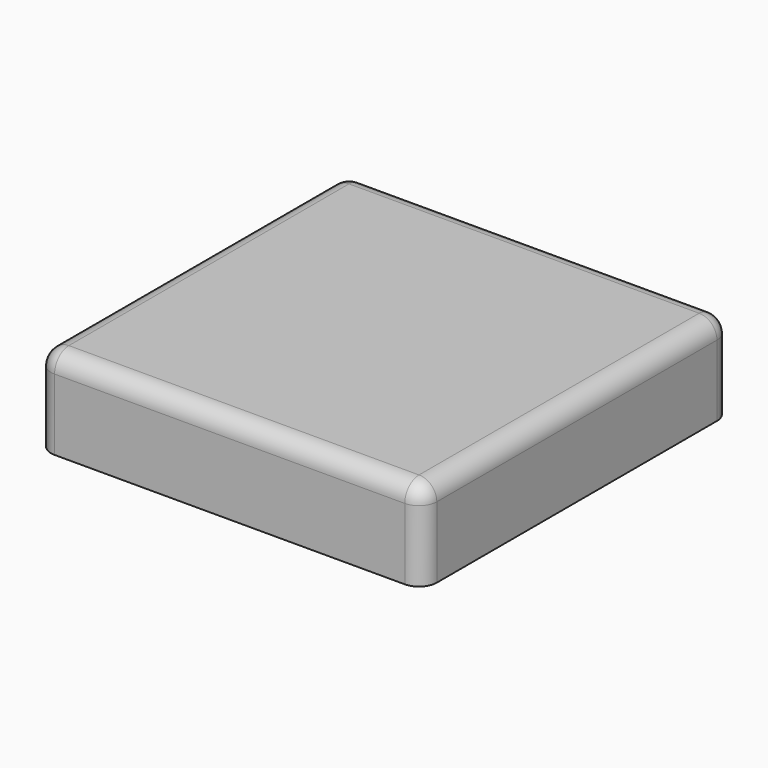
from build123d import *

# Parameters (mm, degrees)
F0_W     = 65
F0_H     = 65
F1_DEPTH = 15
F2_R     = 3
F3_T     = 3


# Not quite as in the source:
# - a shell that OpenCascade refuses in one call is made with other operations: the cavity is built on its own and cut out


with BuildPart() as f1:
    # F0 (on Top) → F1 (new body)
    with BuildSketch(Plane.XY):
        Rectangle(F0_W, F0_H)
    extrude(amount=F1_DEPTH)

    # F2
    f2_edges = [f1.edges().sort_by_distance(p)[0] for p in [
        (0, -32.5, 15),
        (32.5, 0, 15),
        (0, 32.5, 15),
        (-32.5, 0, 15),
        (-32.5, 32.5, 7.5),
        (-32.5, -32.5, 7.5),
        (32.5, 32.5, 7.5),
        (32.5, -32.5, 7.5),
    ]]
    fillet(f2_edges, radius=F2_R)

    # F3: shell of thickness 3, made by hand


with BuildPart() as f3_core1:
    # F3_t2: copy of F1
    add(f1.part)

    # the walls: a layer under each face that stays
    f3_faces = [f3_core1.faces().sort_by_distance(p)[0] for p in [
        (0, -32.5, 6),
        (-32.5, 0, 6),
        (32.5, 0, 6),
        (0, 32.5, 6),
        (0, 0, 15),
    ]]
    thicken(f3_faces, amount=-F3_T, mode=Mode.SUBTRACT)


with BuildPart() as f1_1:
    add(f1.part)

    # what is left inside the walls is the cavity
    f3_cavity = [f3_core1.part.solids().sort_by_distance(p)[0] for p in [
        (0, -9.833333, 0.03),
    ]]
    add(f3_cavity, mode=Mode.SUBTRACT)


solid = f1_1.part
